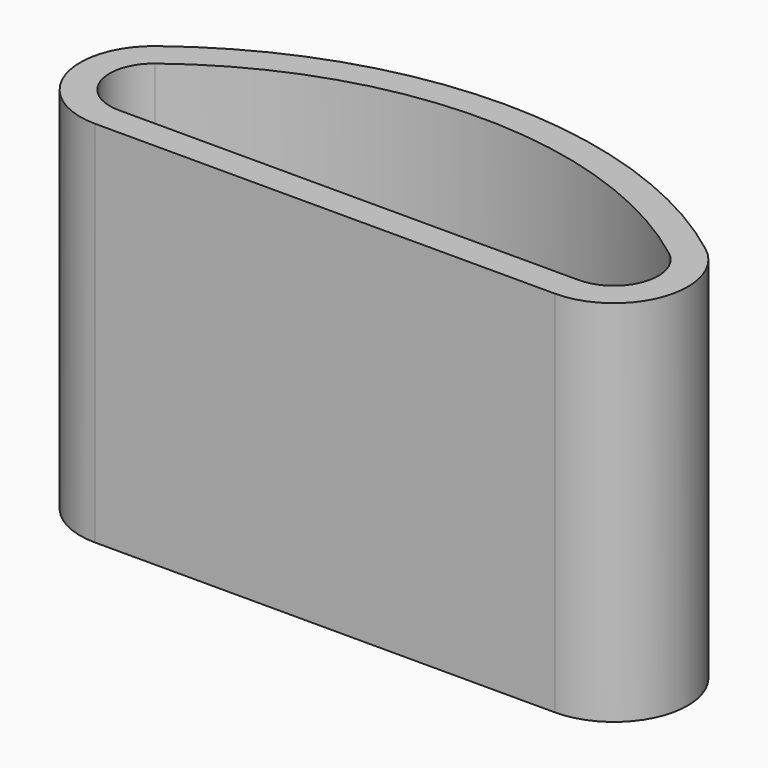
from build123d import *

# Parameters (mm, degrees)
F1_DEPTH = 25
F2_R     = 5
F3_T     = -2


with BuildPart() as f1:
    # F0 (on Top) → F1 (new body)
    with BuildSketch(Plane.XY):
        with BuildLine():
            ThreePointArc((26.5, 0), (0, 15.3), (-26.5, 0))
            Line((-26.5, 0), (26.5, 0))
        make_face()
    extrude(amount=F1_DEPTH)

    # F2
    f2_edges = [f1.edges().sort_by_distance(p)[0] for p in [
        (-26.5, 0, 12.5),
        (26.5, 0, 12.5),
    ]]
    fillet(f2_edges, radius=F2_R)

    # F3
    f3_openings = [f1.faces().sort_by_distance(p)[0] for p in [
        (0, 6.722431, 25),
    ]]
    offset(amount=F3_T, openings=f3_openings)


solid = f1.part
